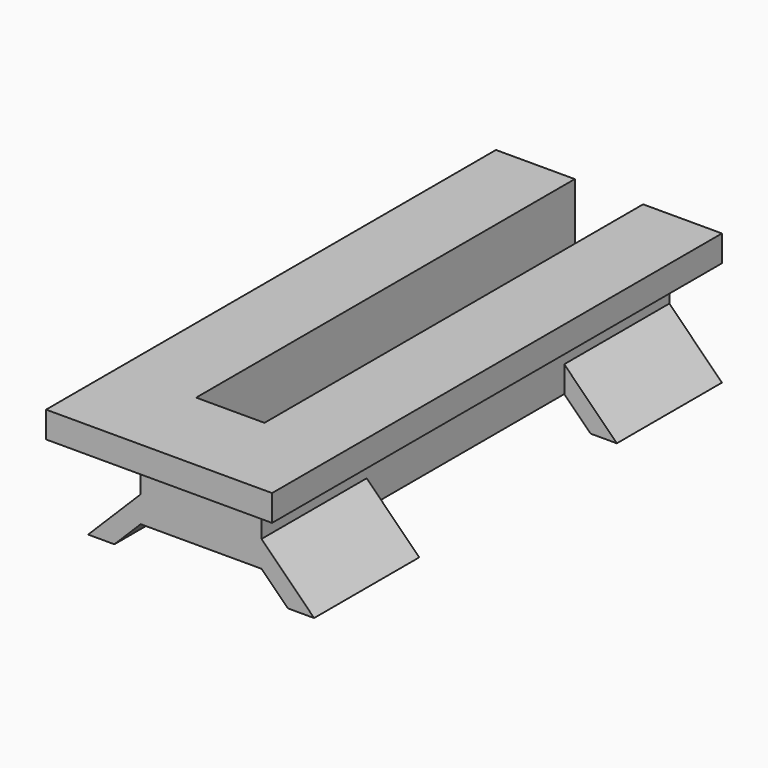
from build123d import *

# Parameters (mm, degrees)
F1_DEPTH      = 2.54
F1_DEPTH_BACK = 2.54
F2_W          = 3.81
F2_H          = 24.638
F2_W_2        = 2.54
F3_DEPTH      = 1.27
F4_W          = 5.715
F4_H          = 2.54
F4_W_2        = 6.35
F6_DEPTH      = 2.54
F5_W          = 6.35
F5_H          = 2.54
F7_DEPTH      = 2.54
F8_T1_DEPTH   = 22.8740361466
F8_T6_DEPTH   = 6.35
F8_T11_DEPTH  = 6.35
F8_T16_DEPTH  = 6.35
F8_T21_DEPTH  = 5.715
F9_W          = 5.842
F9_H          = 1.7639638534
F10_DEPTH     = 1.27
F11_SIZE      = 1.26999


# Not quite as in the source:
# - a fillet or chamfer that OpenCascade refuses, or shapes differently, is made with other operations: its cross-section is extruded or revolved along the edge and cut away or added
# - a fillet or chamfer is up to 0.001 mm smaller than in the source, because OpenCascade refuses the exact size


with BuildPart() as f1:
    # F0 (on Top) → F1 (new body, two sides)
    with BuildSketch(Plane.XY) as f1_sk:
        Polygon((-55.4767026412, 32.9021683285), (-56.7467026412, 32.9021683285), (-56.7467026412, 8.2641683285), (-50.9047026412, 8.2641683285), (-50.9047026412, 32.9021683285), (-52.1747026412, 32.9021683285), (-52.1747026412, 10.0281321819), (-55.4767026412, 10.0281321819), align=None)
    extrude(amount=F1_DEPTH)
    extrude(f1_sk.sketch, amount=-F1_DEPTH_BACK)

    # F2 (on face) → F3 (join)
    with BuildSketch(Plane.XY.offset(2.54)):
        with Locations((-57.3817026412, 20.5831683285)):
            Rectangle(F2_W, F2_H)
        Polygon((-50.9047026412, 8.2641683285), (-55.4767026412, 8.2641683285), (-59.2867026412, 8.2641683285), (-59.2867026412, 5.7241683285), (-48.3647026412, 5.7241683285), (-48.3647026412, 8.2641683285), align=None)
        with Locations((-49.6347026412, 20.5831683285)):
            Rectangle(F2_W_2, F2_H)
        Polygon((-52.1747026412, 10.0281321819), (-55.4767026412, 10.0281321819), (-55.4767026412, 8.2641683285), (-50.9047026412, 8.2641683285), (-50.9047026412, 32.9021683285), (-52.1747026412, 32.9021683285), align=None)
    extrude(amount=F3_DEPTH)

    # F4 (on face) → F6 (join)
    with BuildSketch(Plane(origin=(-56.7467026412, 0, 0), x_dir=(0, -1, 0), z_dir=(-1, 0, 0))):
        with Locations((-30.0446683285, -1.27)):
            Rectangle(F4_W, F4_H)
        with Locations((-11.4391683285, -1.27)):
            Rectangle(F4_W_2, F4_H)
    extrude(amount=F6_DEPTH)

    # F5 (on face) → F7 (join)
    with BuildSketch(Plane.YZ.offset(-50.9047026412)):
        with Locations((29.7271683285, -1.27)):
            Rectangle(F5_W, F5_H)
        with Locations((11.4391683285, -1.27)):
            Rectangle(F5_W, F5_H)
    extrude(amount=F7_DEPTH)

    # F8: chamfer of 2.54 on 6 edges, made by hand

    # F8_s2 → F8_t1 (cut)
    with BuildSketch(Plane.XZ.offset(-32.9021683285)):
        with BuildLine():
            Line((-49.5628605923, -2.611842049), (-52.2465446902, 0.071842049))
            Line((-52.2465446902, 0.071842049), (-52.2973446902, 0.071842049))
            ThreePointArc((-52.2973446902, 0.071842049), (-52.2255026412, -1.2340789755), (-52.2255026412, -2.54))
            Line((-52.2255026412, -2.54), (-52.1747026412, -2.5908))
            ThreePointArc((-52.1747026412, -2.5908), (-50.8687816168, -2.5908), (-49.5628605923, -2.662642049))
            Line((-49.5628605923, -2.662642049), (-49.5628605923, -2.611842049))
        make_face()
        with BuildLine():
            Line((-55.4048605923, 0.071842049), (-58.0885446902, -2.611842049))
            Line((-58.0885446902, -2.611842049), (-58.0885446902, -2.662642049))
            ThreePointArc((-58.0885446902, -2.662642049), (-56.7826236657, -2.5908), (-55.4767026412, -2.5908))
            Line((-55.4767026412, -2.5908), (-55.4259026412, -2.54))
            ThreePointArc((-55.4259026412, -2.54), (-55.4259026412, -1.2340789755), (-55.3540605923, 0.071842049))
            Line((-55.3540605923, 0.071842049), (-55.4048605923, 0.071842049))
        make_face()
    extrude(amount=F8_T1_DEPTH, mode=Mode.SUBTRACT)


with BuildPart() as f8_tool4:
    # F8_s5 → F8_t6 (new body)
    with BuildSketch(Plane.XZ.offset(-32.9021683285)):
        with BuildLine():
            Line((-50.9765446902, 0.071842049), (-48.2928605923, -2.611842049))
            Line((-48.2928605923, -2.611842049), (-48.2420605923, -2.611842049))
            ThreePointArc((-48.2420605923, -2.611842049), (-48.3139026412, -1.3059210245), (-48.3139026412, 0))
            Line((-48.3139026412, 0), (-48.3647026412, 0.0508))
            ThreePointArc((-48.3647026412, 0.0508), (-49.6706236657, 0.0508), (-50.9765446902, 0.122642049))
            Line((-50.9765446902, 0.122642049), (-50.9765446902, 0.071842049))
        make_face()
    extrude(amount=F8_T6_DEPTH)

    split(bisect_by=Plane.YZ.offset(-50.9047026412), keep=Keep.TOP)


with BuildPart() as f1_1:
    add(f1.part)

    # F8_t3: cut F8_tool4
    add(f8_tool4.part, mode=Mode.SUBTRACT)


with BuildPart() as f8_tool9:
    # F8_s10 → F8_t11 (new body)
    with BuildSketch(Plane.XZ.offset(-14.6141683285)):
        with BuildLine():
            Line((-50.9765446902, 0.071842049), (-48.2928605923, -2.611842049))
            Line((-48.2928605923, -2.611842049), (-48.2420605923, -2.611842049))
            ThreePointArc((-48.2420605923, -2.611842049), (-48.3139026412, -1.3059210245), (-48.3139026412, 0))
            Line((-48.3139026412, 0), (-48.3647026412, 0.0508))
            ThreePointArc((-48.3647026412, 0.0508), (-49.6706236657, 0.0508), (-50.9765446902, 0.122642049))
            Line((-50.9765446902, 0.122642049), (-50.9765446902, 0.071842049))
        make_face()
    extrude(amount=F8_T11_DEPTH)

    split(bisect_by=Plane.YZ.offset(-50.9047026412), keep=Keep.TOP)


with BuildPart() as f1_2:
    add(f1_1.part)

    # F8_t8: cut F8_tool9
    add(f8_tool9.part, mode=Mode.SUBTRACT)


with BuildPart() as f8_tool14:
    # F8_s15 → F8_t16 (new body)
    with BuildSketch(Plane.XZ.offset(-8.2641683285)):
        with BuildLine():
            Line((-56.6748605923, 0.071842049), (-59.3585446902, -2.611842049))
            Line((-59.3585446902, -2.611842049), (-59.4093446902, -2.611842049))
            ThreePointArc((-59.4093446902, -2.611842049), (-59.3375026412, -1.3059210245), (-59.3375026412, 0))
            Line((-59.3375026412, 0), (-59.2867026412, 0.0508))
            ThreePointArc((-59.2867026412, 0.0508), (-57.9807816168, 0.0508), (-56.6748605923, 0.122642049))
            Line((-56.6748605923, 0.122642049), (-56.6748605923, 0.071842049))
        make_face()
    extrude(amount=-F8_T16_DEPTH)

    split(bisect_by=Plane.YZ.offset(-56.7467026412), keep=Keep.BOTTOM)


with BuildPart() as f1_3:
    add(f1_2.part)

    # F8_t13: cut F8_tool14
    add(f8_tool14.part, mode=Mode.SUBTRACT)


with BuildPart() as f8_tool19:
    # F8_s20 → F8_t21 (new body)
    with BuildSketch(Plane.XZ.offset(-27.1871683285)):
        with BuildLine():
            Line((-56.6748605923, 0.071842049), (-59.3585446902, -2.611842049))
            Line((-59.3585446902, -2.611842049), (-59.4093446902, -2.611842049))
            ThreePointArc((-59.4093446902, -2.611842049), (-59.3375026412, -1.3059210245), (-59.3375026412, 0))
            Line((-59.3375026412, 0), (-59.2867026412, 0.0508))
            ThreePointArc((-59.2867026412, 0.0508), (-57.9807816168, 0.0508), (-56.6748605923, 0.122642049))
            Line((-56.6748605923, 0.122642049), (-56.6748605923, 0.071842049))
        make_face()
    extrude(amount=-F8_T21_DEPTH)

    split(bisect_by=Plane.YZ.offset(-56.7467026412), keep=Keep.BOTTOM)


with BuildPart() as f1_4:
    add(f1_3.part)

    # F8_t18: cut F8_tool19
    add(f8_tool19.part, mode=Mode.SUBTRACT)

    # F9 (on face) → F10 (cut)
    with BuildSketch(Plane(origin=(0, 0, -2.54), x_dir=(1, 0, 0), z_dir=(0, 0, -1))):
        with Locations((-53.8257026412, -9.1461502552)):
            Rectangle(F9_W, F9_H)
    extrude(amount=-F10_DEPTH, mode=Mode.SUBTRACT)

    # F11 (size 1.27 in the source; OpenCascade refuses exactly that, so slightly less here)
    f11_edges = [f1_4.edges().sort_by_distance(p)[0] for p in [
        (-50.904703, 9.14615, -2.54),
        (-56.746703, 9.14615, -2.54),
    ]]
    chamfer(f11_edges, length=F11_SIZE)


solid = f1_4.part
